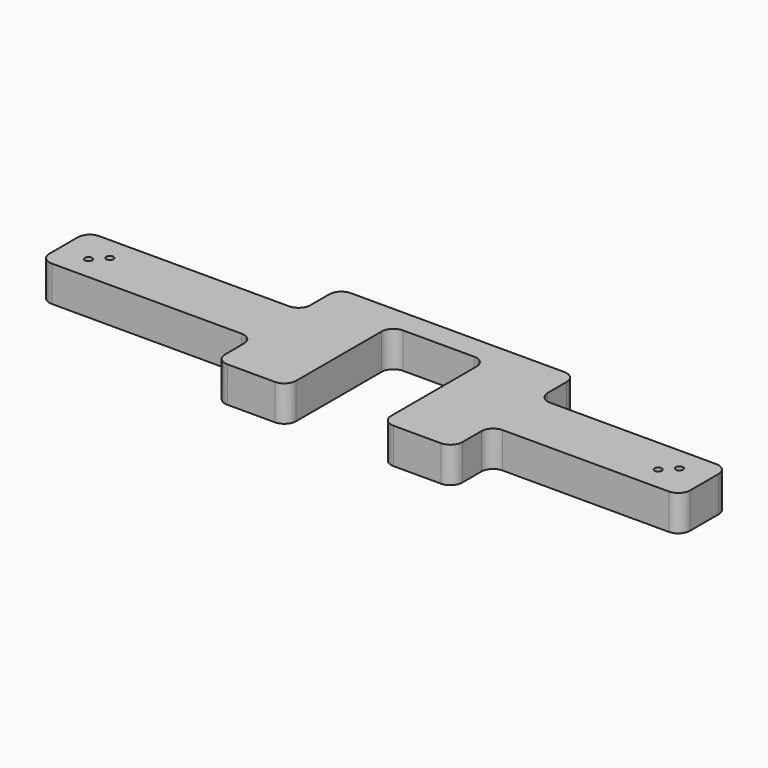
from build123d import *

# Parameters (mm, degrees)
F1_DEPTH  = 150
F2_R      = 50
F3_W      = 150
F3_H      = 150
F4_DEPTH  = 10
F6_R      = 15
F7_DEPTH  = 200
F8_R      = 15
F9_DEPTH  = 200
F10_W     = 25
F10_H     = 50
F11_DEPTH = 60
F12_W     = 25
F12_H     = 40
F13_DEPTH = 100
F14_W     = 25
F14_H     = 40
F15_DEPTH = 100
F16_W     = 25
F16_H     = 40
F17_DEPTH = 1000


# Not quite as in the source:
# - two fillets or chamfers of one size are made in one step
# - a feature names something its author has since deleted; it is built from what else it names


with BuildPart() as f1:
    # F0 (on Top) → F1 (new body)
    with BuildSketch(Plane.XY):
        Polygon((0, 250), (0, 0), (900, 0), (900, -200), (1200, -200), (1200, 350), (1600, 350), (1600, -200), (1900, -200), (1900, 0), (2700, 0), (2700, 250), (1900, 250), (1900, 450), (900, 450), (900, 250), align=None)
    extrude(amount=F1_DEPTH)

    # F2
    f2_edges = [f1.edges().sort_by_distance(p)[0] for p in [
        (1600, 350, 75),
        (1600, -200, 75),
        (1900, -200, 75),
        (1900, 450, 75),
        (900, 450, 75),
        (900, 250, 75),
        (0, 250, 75),
        (0, 0, 75),
        (900, 0, 75),
        (900, -200, 75),
        (1200, -200, 75),
        (1200, 350, 75),
        (1900, 0, 75),
        (2700, 0, 75),
        (2700, 250, 75),
        (1900, 250, 75),
    ]]
    fillet(f2_edges, radius=F2_R)

    # F3 (on face) → F4 (cut)
    with BuildSketch(Plane(origin=(0, 0, 0), x_dir=(1, 0, 0), z_dir=(0, 0, -1))):
        with Locations((150, -125)):
            Rectangle(F3_W, F3_H)
        with Locations((2550, -125)):
            Rectangle(F3_W, F3_H)
    extrude(amount=-F4_DEPTH, mode=Mode.SUBTRACT)

    # F6 (on face) → F7 (cut)
    with BuildSketch(Plane(origin=(0, 0, 10), x_dir=(1, 0, 0), z_dir=(0, 0, -1))):
        with Locations((175, -150)):
            Circle(F6_R)
        with Locations((125, -100)):
            Circle(F6_R)
    extrude(amount=-F7_DEPTH, mode=Mode.SUBTRACT)

    # F8 (on face) → F9 (cut)
    with BuildSketch(Plane(origin=(0, 0, 10), x_dir=(1, 0, 0), z_dir=(0, 0, -1))):
        with Locations((2525, -100)):
            Circle(F8_R)
        with Locations((2575, -150)):
            Circle(F8_R)
    extrude(amount=-F9_DEPTH, mode=Mode.SUBTRACT)

    # F10 (on face) → F11 (join)
    with BuildSketch(Plane(origin=(0, 0, 0), x_dir=(1, 0, 0), z_dir=(0, 0, -1))):
        with Locations((1077.5, 75)):
            Rectangle(F10_W, F10_H)
        with Locations((1722.5, 75)):
            Rectangle(F10_W, F10_H)
        with Locations((1077.5, -325)):
            Rectangle(F10_W, F10_H)
        with Locations((1722.5, -325)):
            Rectangle(F10_W, F10_H)
    extrude(amount=F11_DEPTH)

    # F12 (on face) → F13 (cut)
    with BuildSketch(Plane(origin=(1065, 0, 0), x_dir=(0, -1, 0), z_dir=(-1, 0, 0))):
        with Locations((87.5, -20)):
            Rectangle(F12_W, F12_H)
    extrude(amount=-F13_DEPTH, mode=Mode.SUBTRACT)

    # F14 (on face) → F15 (cut)
    with BuildSketch(Plane(origin=(1710, 0, 0), x_dir=(0, -1, 0), z_dir=(-1, 0, 0))):
        with Locations((87.5, -20)):
            Rectangle(F14_W, F14_H)
    extrude(amount=-F15_DEPTH, mode=Mode.SUBTRACT)

    # F16 (on face) → F17 (cut)
    with BuildSketch(Plane(origin=(1065, 0, 0), x_dir=(0, -1, 0), z_dir=(-1, 0, 0))):
        with Locations((-312.5, -20)):
            Rectangle(F16_W, F16_H)
    extrude(amount=-F17_DEPTH, mode=Mode.SUBTRACT)


solid = f1.part
